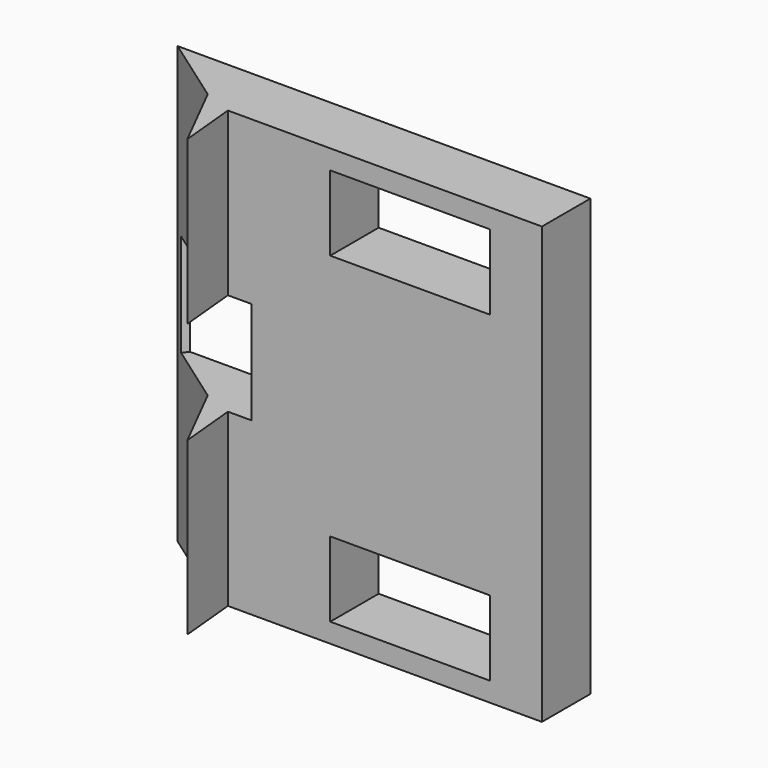
from build123d import *

# Parameters (mm, degrees)
F0_W     = 135
F0_H     = 180
F1_DEPTH = 25
F3_DEPTH = 180
F4_W     = 51.5650697052
F4_H     = 42.2876738012
F5_DEPTH = 25
F6_W     = 66.04
F6_H     = 31
F7_DEPTH = 25
F8_W     = 32.0292665178
F8_H     = 42.2876738012
F9_DEPTH = 10


# Not quite as in the source:
# - a feature names something its author has since deleted; it is built from what else it names


with BuildPart() as f1:
    # F0 (on Front) → F1 (new body)
    with BuildSketch(Plane.XZ):
        Rectangle(F0_W, F0_H)
    extrude(amount=F1_DEPTH)

    # F2 (on face) → F3 (join)
    with BuildSketch(Plane(origin=(0, 0, -90), x_dir=(1, 0, 0), z_dir=(0, 0, -1))):
        Polygon((-74.269764297, 20.2139050914), (-67.5, 25), (-62.1096342802, 25), (-59.8334595561, 48.8052852452), align=None)
        Polygon((-67.5, 0), (-67.5, 25), (-74.269764297, 20.2139050914), (-102.8616279364, 0), align=None)
    extrude(amount=-F3_DEPTH)

    # F4 (on face) → F5 (cut)
    with BuildSketch(Plane(origin=(-34.2790786746, -48.4865610438, 0), x_dir=(0.8165449841, -0.5772818107, 0), z_dir=(-0.5772818107, -0.8165449841, 0))):
        with Locations((-54.0774967521, 1.7260275781)):
            Rectangle(F4_W, F4_H)
    extrude(amount=-F5_DEPTH, mode=Mode.SUBTRACT)

    # F6 (on face) → F7 (cut)
    with BuildSketch(Plane.XZ.offset(25)):
        with Locations((13.1429424509, 66.5)):
            Rectangle(F6_W, F6_H)
        with Locations((13.1429424509, -66.5)):
            Rectangle(F6_W, F6_H)
    extrude(amount=-F7_DEPTH, mode=Mode.SUBTRACT)

    # F8 (on face) → F9 (cut)
    with BuildSketch(Plane(origin=(-67.3147543785, -33.9884364638, 0), x_dir=(0.4507223021, -0.8926642181, 0), z_dir=(-0.8926642181, -0.4507223021, 0))):
        with Locations((0.5838238992, 1.7260275781)):
            Rectangle(F8_W, F8_H)
    extrude(amount=-F9_DEPTH, mode=Mode.SUBTRACT)


solid = f1.part
